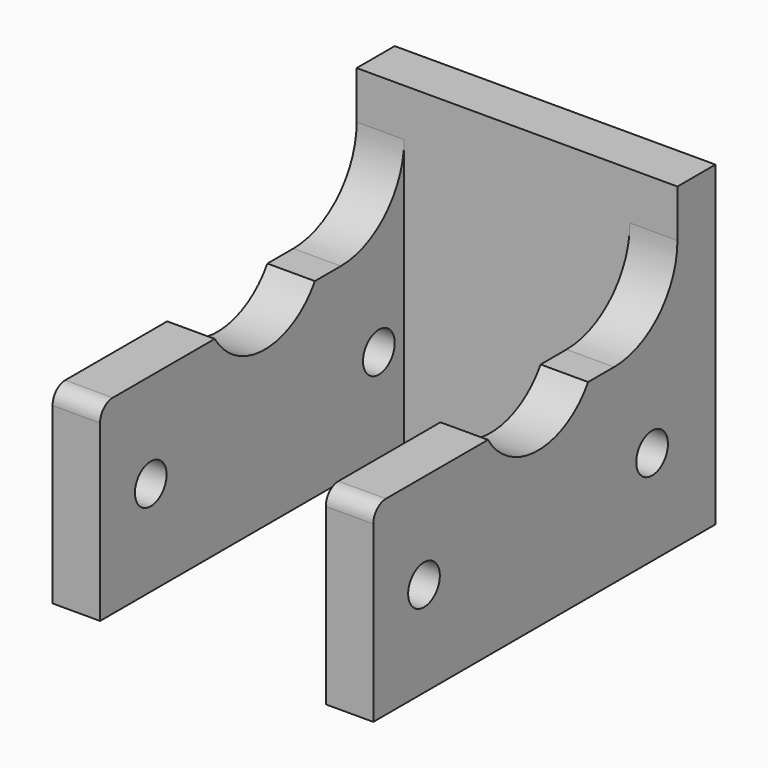
from build123d import *

# Parameters (mm, degrees)
F0_W     = 3
F0_H     = 24
F1_DEPTH = 12
F2_R     = 1.25
F3_DEPTH = 150
F4_DEPTH = 20
F5_R     = 5
F6_R     = 1
F7_DEPTH = 150


# Not quite as in the source:
# - a feature names something its author has since deleted; it is built from what else it names


with BuildPart() as f1:
    # F0 (on Top) → F1 (new body)
    with BuildSketch(Plane.XY):
        with Locations((8.625, -1.5)):
            Rectangle(F0_W, F0_H)
        with Locations((-8.625, -1.5)):
            Rectangle(F0_W, F0_H)
        Polygon((10.125, 13.5), (-10.125, 13.5), (-10.125, 10.5), (-7.125, 10.5), (7.125, 10.5), (10.125, 10.5), align=None)
    extrude(amount=F1_DEPTH)

    # F2 (on face) → F3 (cut)
    with BuildSketch(Plane.YZ.offset(10.125)):
        with Locations((-9.5, 6)):
            Circle(F2_R)
        with Locations((8.5, 6)):
            Circle(F2_R)
    extrude(amount=-F3_DEPTH, mode=Mode.SUBTRACT)

    # F0 (on Top) → F4 (join)
    with BuildSketch(Plane.XY):
        Polygon((10.125, 13.5), (-10.125, 13.5), (-10.125, 10.5), (-7.125, 10.5), (7.125, 10.5), (10.125, 10.5), align=None)
    extrude(amount=F4_DEPTH)

    # F5
    f5_edges = [f1.edges().sort_by_distance(p)[0] for p in [
        (8.625, 10.5, 12),
        (-8.625, 10.5, 12),
    ]]
    fillet(f5_edges, radius=F5_R)

    # F6
    f6_edges = [f1.edges().sort_by_distance(p)[0] for p in [
        (8.625, -13.5, 12),
        (-8.625, -13.5, 12),
    ]]
    fillet(f6_edges, radius=F6_R)

    # F2 (on face) → F7 (cut)
    with BuildSketch(Plane.YZ.offset(10.125)):
        with BuildLine():
            ThreePointArc((-4.4522145691, 12), (-0.5, 9.8), (3.4522145691, 12))
            Line((3.4522145691, 12), (-4.4522145691, 12))
        make_face()
    extrude(amount=-F7_DEPTH, mode=Mode.SUBTRACT)


solid = f1.part
